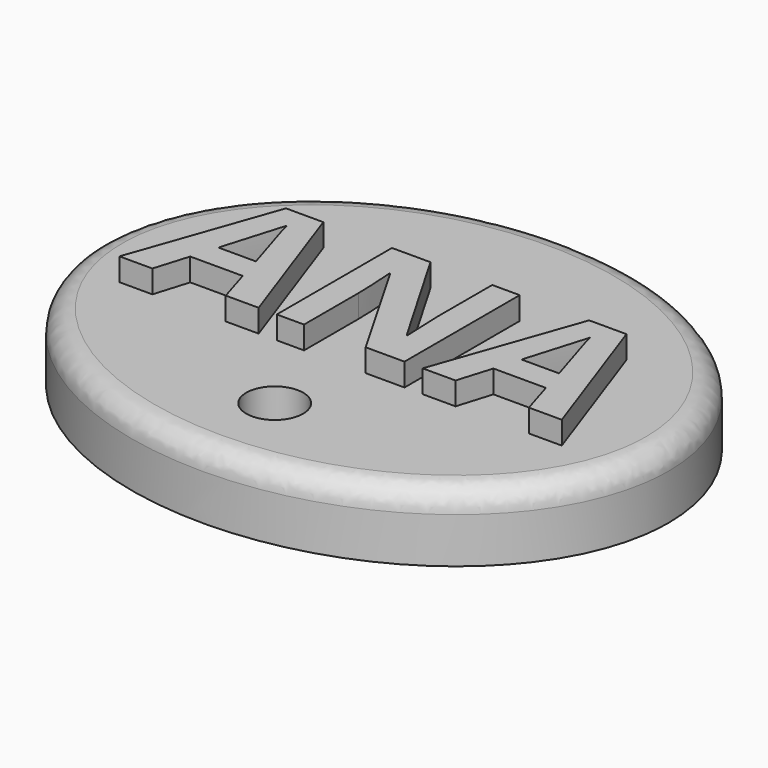
from build123d import *

# Parameters (mm, degrees)
F1_DEPTH     = 6
F2_TEXT_SIZE = 17.7162629758
F3_DEPTH     = 2
F4_R         = 2


# Not quite as in the source:
# - Text() gives the source's letters only with a copy of the font that has no kerning and outlines rounded to 1/6400 em; it was checked with that copy


with BuildPart() as f1:
    # F0 (on Top) → F1 (new body)
    with BuildSketch(Plane.XY):
        with BuildLine():
            add(Edge.make_bspline(
                [(-14.6254315045, -20), (10.3745684955, -20), (10.3745684955, 0)],
                knots=[4.7123889804, 4.7123889804, 4.7123889804, 6.2831853072, 6.2831853072, 6.2831853072], degree=2, weights=[1, 0.7071067812, 1]))
            add(Edge.make_bspline(
                [(10.3745684955, 0), (10.3745684955, 48.2842712475), (-32.3031010342, 14.1421356237), (-74.9807705638, -20), (-14.6254315045, -20)],
                knots=[0, 0, 0, 2.3561944902, 2.3561944902, 4.7123889804, 4.7123889804, 4.7123889804], degree=2, weights=[1, 0.3826834324, 1, 0.3826834324, 1]))
        make_face()
        with BuildLine():
            ThreePointArc((-12.1254315045, -12), (-12.8576645515, -13.767766953), (-14.6254315045, -14.5))
            ThreePointArc((-14.6254315045, -14.5), (-16.3931984575, -10.232233047), (-12.1254315045, -12))
        make_face(mode=Mode.SUBTRACT)
    extrude(amount=F1_DEPTH)

    # F2 (on face) → F3 (join)
    with BuildSketch(Plane.XY.offset(6)):
        with Locations((-34.1657345138, -4.6210228814)):
            Text('ANA', F2_TEXT_SIZE, font='Open Sans', font_style=FontStyle.BOLD, text_align=(TextAlign.LEFT, TextAlign.BOTTOM))
    extrude(amount=F3_DEPTH)

    # F4
    f4_edges = [f1.edges().sort_by_distance(p)[0] for p in [
        (-31.308789, 14.895166, 6),
    ]]
    fillet(f4_edges, radius=F4_R)


solid = f1.part
